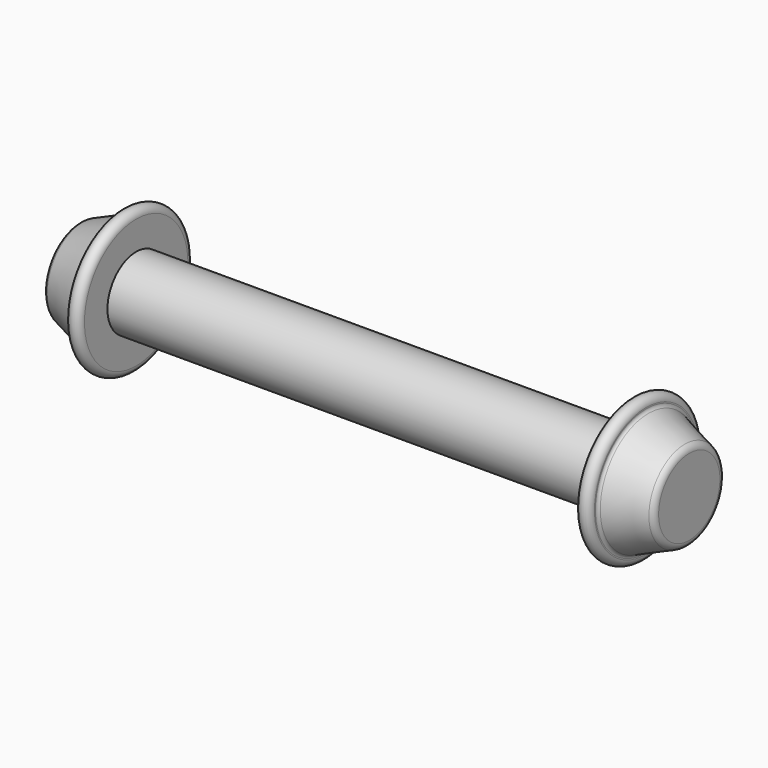
from build123d import *

# Parameters (mm, degrees)
F0_W = 34.5
F0_H = 5


# Not quite as in the source:
# - ends of sketch curves that miss each other by under 0.0002 mm in the source are joined


with BuildPart() as f1:
    # F0 (on Front) → F1 (revolve)
    with BuildSketch(Plane.XZ):
        with BuildLine():
            Line((-34.5, -388.122387), (-34.5, -383.122387))
            Line((-34.5, -383.122387), (-34.5, -379.122387))
            ThreePointArc((-34.5, -379.122387), (-35.5, -378.122387), (-36.5, -379.122387))
            Line((-36.5, -379.122387), (-36.5, -379.289054))
            ThreePointArc((-36.5, -379.289054), (-36.5839747248, -379.5664039061), (-36.8076918817, -379.750592284))
            Line((-36.8076918817, -379.750592284), (-41.884615, -381.865977))
            ThreePointArc((-41.884615, -381.865977), (-42.3320501877, -382.2343536438), (-42.5, -382.789054))
            Line((-42.5, -382.789054), (-42.5, -388.122387))
            Line((-42.5, -388.122387), (-34.5, -388.122387))
        make_face()
        with Locations((-17.25, -385.622387)):
            Rectangle(F0_W, F0_H)
    revolve(axis=Axis((-21.25, 0, -388.122387), (-1, 0, 0)))

    # F2: F1 across face


with BuildPart() as f1_1:
    add(f1.part)
    add(f1.part.mirror(Plane(origin=(0, 0, -388.122387), x_dir=(0, 1, 0), z_dir=(1, 0, 0))))


solid = f1_1.part
